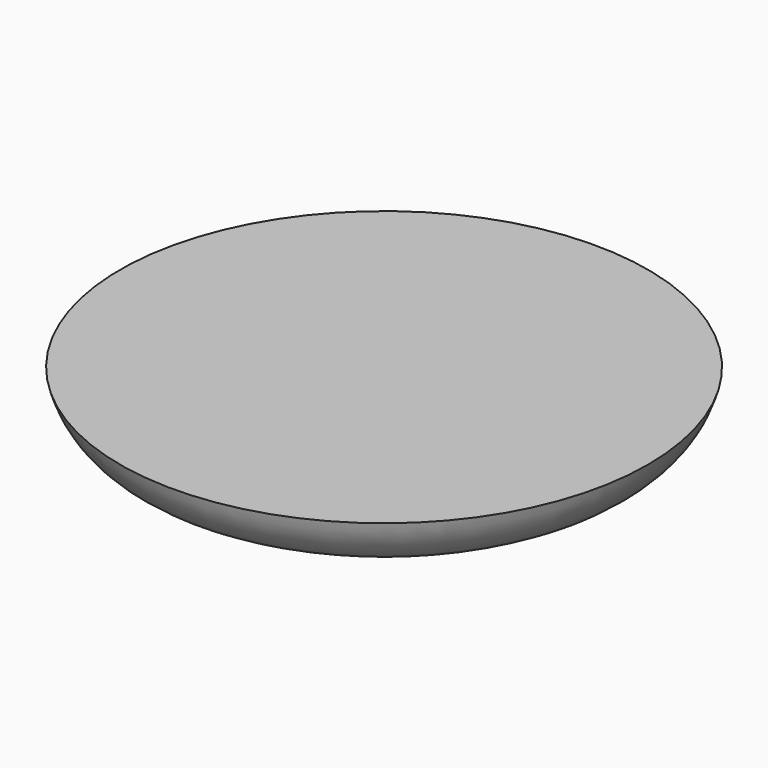
from build123d import *

# Parameters (mm, degrees)
F0_R     = 16.9278894976
F1_DEPTH = 3.81


# Not quite as in the source:
# - a fillet or chamfer that OpenCascade refuses, or shapes differently, is made with other operations: its cross-section is extruded or revolved along the edge and cut away or added


with BuildPart() as f1:
    # F0 (on Top) → F1 (new body)
    with BuildSketch(Plane.XY):
        Circle(F0_R)
    extrude(amount=F1_DEPTH)

    # F2: fillet of radius 5.08 on 1 edges, made by hand

    # F2_s1 → F2_t2 (revolve, cut)
    with BuildSketch(Plane.XZ):
        with BuildLine():
            ThreePointArc((16.9278894976, 3.81), (15.1200526212, 1.0639073716), (12.0092006479, 0))
            Line((12.0092006479, 0), (16.9278894976, 0))
            Line((16.9278894976, 0), (16.9278894976, 3.81))
        make_face()
    revolve(axis=Axis((0, 0, 0), (0, 0, 1)), mode=Mode.SUBTRACT)


solid = f1.part
